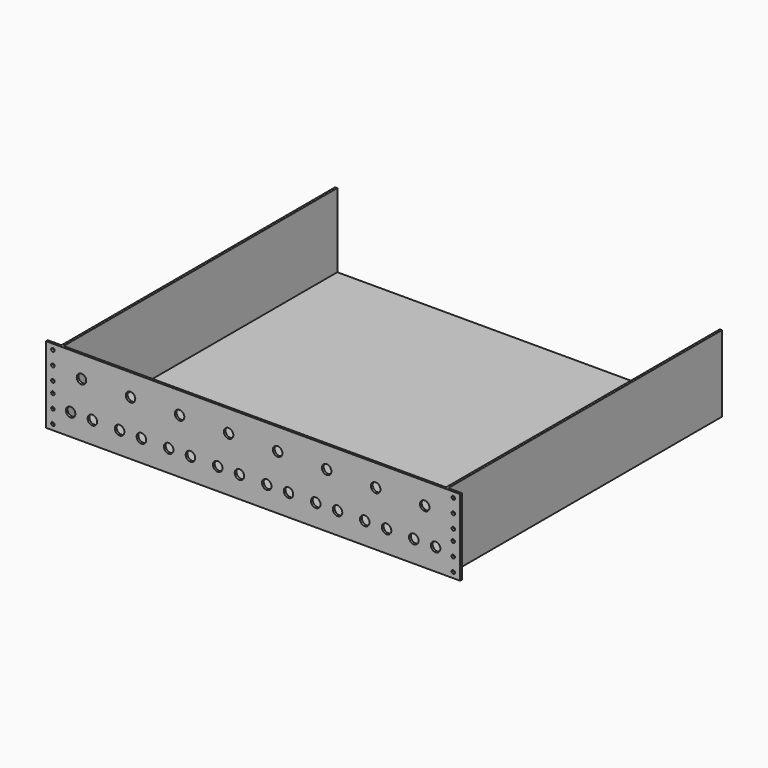
from build123d import *

# Parameters (mm, degrees)
F0_W        = 482.6
F0_H        = 88.9
F0_R        = 5.5372
F1_DEPTH    = 2.54
F2_W        = 450.85
F2_H        = 88.9
F3_DEPTH    = 398.78
F4_DEPTH    = 398.781
F6_D        = 4.0386
F7_T        = 2.54
F7_T3_DEPTH = 93.98


# Not quite as in the source:
# - a shell that OpenCascade refuses in one call is made with other operations: the cavity is built on its own and cut out


with BuildPart() as f1:
    # F0 (on Front) → F1 (new body)
    with BuildSketch(Plane.XZ):
        Rectangle(F0_W, F0_H)
        with Locations((-212.725, -19.05)):
            Circle(F0_R, mode=Mode.SUBTRACT)
        with Locations((-187.325, -19.05)):
            Circle(F0_R, mode=Mode.SUBTRACT)
        with Locations((-155.575, -19.05)):
            Circle(F0_R, mode=Mode.SUBTRACT)
        with Locations((-130.175, -19.05)):
            Circle(F0_R, mode=Mode.SUBTRACT)
        with Locations((-98.425, -19.05)):
            Circle(F0_R, mode=Mode.SUBTRACT)
        with Locations((-73.025, -19.05)):
            Circle(F0_R, mode=Mode.SUBTRACT)
        with Locations((-41.275, -19.05)):
            Circle(F0_R, mode=Mode.SUBTRACT)
        with Locations((-15.875, -19.05)):
            Circle(F0_R, mode=Mode.SUBTRACT)
        with Locations((15.875, -19.05)):
            Circle(F0_R, mode=Mode.SUBTRACT)
        with Locations((41.275, -19.05)):
            Circle(F0_R, mode=Mode.SUBTRACT)
        with Locations((73.025, -19.05)):
            Circle(F0_R, mode=Mode.SUBTRACT)
        with Locations((98.425, -19.05)):
            Circle(F0_R, mode=Mode.SUBTRACT)
        with Locations((130.175, -19.05)):
            Circle(F0_R, mode=Mode.SUBTRACT)
        with Locations((155.575, -19.05)):
            Circle(F0_R, mode=Mode.SUBTRACT)
        with Locations((187.325, -19.05)):
            Circle(F0_R, mode=Mode.SUBTRACT)
        with Locations((212.725, -19.05)):
            Circle(F0_R, mode=Mode.SUBTRACT)
        with Locations((-200.025, 19.05)):
            Circle(F0_R, mode=Mode.SUBTRACT)
        with Locations((-142.875, 19.05)):
            Circle(F0_R, mode=Mode.SUBTRACT)
        with Locations((-85.725, 19.05)):
            Circle(F0_R, mode=Mode.SUBTRACT)
        with Locations((-28.575, 19.05)):
            Circle(F0_R, mode=Mode.SUBTRACT)
        with Locations((28.575, 19.05)):
            Circle(F0_R, mode=Mode.SUBTRACT)
        with Locations((85.725, 19.05)):
            Circle(F0_R, mode=Mode.SUBTRACT)
        with Locations((142.875, 19.05)):
            Circle(F0_R, mode=Mode.SUBTRACT)
        with Locations((200.025, 19.05)):
            Circle(F0_R, mode=Mode.SUBTRACT)
    extrude(amount=F1_DEPTH)

    # F2 (on face) → F3 (join)
    with BuildSketch(Plane(origin=(0, 0, 0), x_dir=(-1, 0, 0), z_dir=(0, 1, 0))):
        Rectangle(F2_W, F2_H)
    extrude(amount=F3_DEPTH)

    # F4 (cut, through all): faces of the model
    f4_faces = [f1.faces().sort_by_distance(p)[0] for p in [
        (-200.025, 0, 19.05),
        (-212.725, 0, -19.05),
        (-187.325, 0, -19.05),
        (-142.875, 0, 19.05),
        (-155.575, 0, -19.05),
        (-130.175, 0, -19.05),
        (-85.725, 0, 19.05),
        (-98.425, 0, -19.05),
        (-73.025, 0, -19.05),
        (-41.275, 0, -19.05),
        (-28.575, 0, 19.05),
        (-15.875, 0, -19.05),
        (15.875, 0, -19.05),
        (28.575, 0, 19.05),
        (41.275, 0, -19.05),
        (73.025, 0, -19.05),
        (85.725, 0, 19.05),
        (98.425, 0, -19.05),
        (130.175, 0, -19.05),
        (142.875, 0, 19.05),
        (155.575, 0, -19.05),
        (187.325, 0, -19.05),
        (200.025, 0, 19.05),
        (212.725, 0, -19.05),
    ]]
    extrude(f4_faces, amount=-F4_DEPTH, mode=Mode.SUBTRACT)

    # F6 (through all)
    with Locations(Plane.XZ.offset(2.54)):
        with Locations((233.3625, -38.1), (233.3625, -6.35), (-233.3625, 22.225), (233.3625, -22.225), (-233.3625, 38.1), (-233.3625, 6.35), (-233.3625, -22.225), (-233.3625, -6.35), (-233.3625, -38.1), (233.3625, 38.1), (233.3625, 22.225), (233.3625, 6.35)):
            Hole(F6_D / 2)

    # F7: shell of thickness 2.54, made by hand


with BuildPart() as f7_core1:
    # F7_t2: copy of F1
    add(f1.part)

    # the walls: a layer under each face that stays
    f7_faces = [f7_core1.faces().sort_by_distance(p)[0] for p in [
        (241.3, -1.27, 0),
        (0, -2.54, 0),
        (-241.3, -1.27, 0),
        (-233.3625, 0, 0),
        (-225.425, 199.39, 0),
        (225.425, 199.39, 0),
        (233.3625, 0, 0),
        (0, 198.12, -44.45),
        (-235.3818, -1.27, -38.1),
        (-235.3818, -1.27, -22.225),
        (-235.3818, -1.27, -6.35),
        (231.3432, -1.27, -38.1),
        (231.3432, -1.27, -22.225),
        (231.3432, -1.27, -6.35),
        (-235.3818, -1.27, 6.35),
        (-235.3818, -1.27, 22.225),
        (-235.3818, -1.27, 38.1),
        (231.3432, -1.27, 6.35),
        (231.3432, -1.27, 22.225),
        (231.3432, -1.27, 38.1),
    ]]
    thicken(f7_faces, amount=-F7_T, mode=Mode.SUBTRACT)

    # F7_s4 → F7_t3 (cut)
    with BuildSketch(Plane.XY.offset(-46.99)):
        Polygon((-225.4504, 0.0254), (-225.425, -2.54), (-222.885, -2.54), (-222.885, 0), align=None)
        Polygon((225.4504, 0.0254), (222.885, 0), (222.885, -2.54), (225.425, -2.54), align=None)
    extrude(amount=F7_T3_DEPTH, mode=Mode.SUBTRACT)


with BuildPart() as f1_1:
    add(f1.part)

    # what is left inside the walls is the cavity
    f7_cavity = [f7_core1.part.solids().sort_by_distance(p)[0] for p in [
        (0, 132.926667, 44.4246),
    ]]
    add(f7_cavity, mode=Mode.SUBTRACT)


solid = f1_1.part
